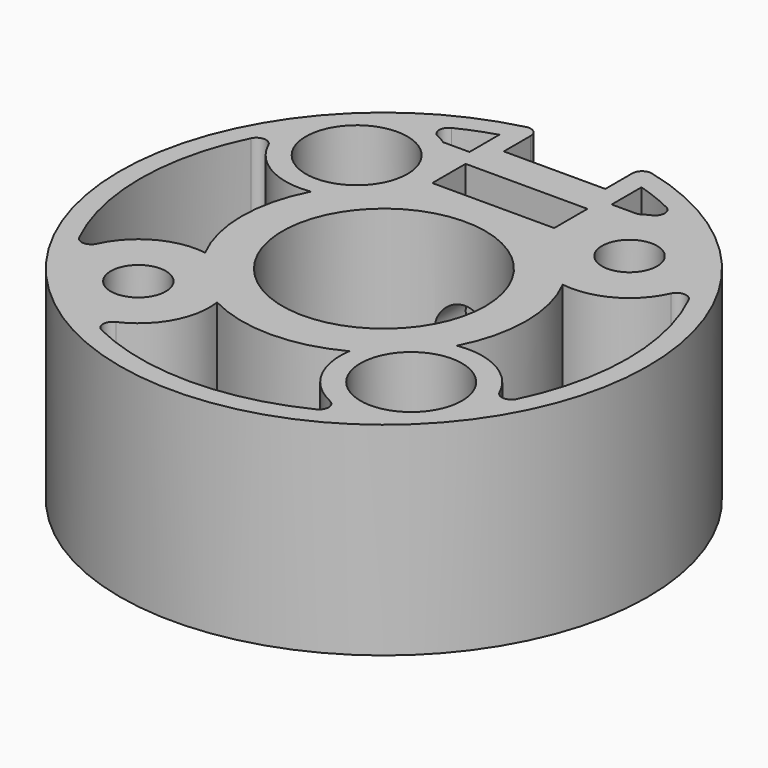
from build123d import *

# Parameters (mm, degrees)
F0_R             = 2.15265
F0_R_2           = 7.9375
F1_DEPTH         = 15.875
F2_R             = 2.15265
F3_REACH         = 43.3958636501
F6_R             = 3.96875
F7_DEPTH         = 12.7
F8_R             = 3.96875
F9_DEPTH         = 12.7
F11_DEPTH        = 15.875
F11_COPIES_COUNT = 3
F11_COPIES_ANGLE = 180
F12_R            = 2.15265
F13_REACH        = 43.3958636501
F15_DEPTH        = 15.875
F16_R            = 0.762


# Not quite as in the source:
# - a pattern or mirror of a feature is missing from the dataset's text; its kind, count and spacing are read off the source's solid


with BuildPart() as f1:
    # F0 (on Top) → F1 (new body)
    with BuildSketch(Plane.XY):
        with BuildLine():
            Line((3.96875, 16.66875), (0, 16.66875))
            Line((0, 16.66875), (-3.96875, 16.66875))
            Line((-3.96875, 16.66875), (-3.96875, 20.2522944302))
            ThreePointArc((-3.96875, 20.2522944302), (0, -20.6375), (3.96875, 20.2522944302))
            Line((3.96875, 20.2522944302), (3.96875, 16.66875))
        make_face()
        with Locations((-10.6640541438, -10.6640541438)):
            Circle(F0_R, mode=Mode.SUBTRACT)
        with Locations((10.6640541438, -10.6640541438)):
            Circle(F0_R, mode=Mode.SUBTRACT)
        with Locations((-10.6640541438, 10.6640541438)):
            Circle(F0_R, mode=Mode.SUBTRACT)
        Circle(F0_R_2, mode=Mode.SUBTRACT)
        Polygon((-4.7625, 13.928725), (0, 13.928725), (4.7625, 13.928725), (4.7625, 10.677525), (-4.7625, 10.677525), align=None, mode=Mode.SUBTRACT)
        with Locations((10.6640541438, 10.6640541438)):
            Circle(F0_R, mode=Mode.SUBTRACT)
    extrude(amount=F1_DEPTH)

    f3_end = f1.faces().sort_by_distance((-7.9375, 0, 7.9375))[0]
    # F2 (on face) → F3 (cut, up to a face of the model that its end follows)
    with BuildSketch(Plane(origin=(0, 16.66875, 0), x_dir=(-1, 0, 0), z_dir=(0, 1, 0))):
        with Locations((0, 7.9375)):
            Circle(F2_R)
    f3_long = extrude(amount=-F3_REACH, mode=Mode.PRIVATE)
    add(split(f3_long, bisect_by=f3_end, keep=Keep.ALL, mode=Mode.PRIVATE).solids().sort_by_distance((0, 16.66875, 7.9375))[0], mode=Mode.SUBTRACT)

    # F6 (on face) → F7 (cut, through all)
    with BuildSketch(Plane.XY.offset(15.875)):
        with Locations((-10.6640541438, 10.6640541438)):
            Circle(F6_R)
        with Locations((10.6640541438, -10.6640541438)):
            Circle(F6_R)
    extrude(amount=-F7_DEPTH, mode=Mode.SUBTRACT)

    # F8 (on face) → F9 (cut, through all)
    with BuildSketch(Plane(origin=(0, 0, 0), x_dir=(1, 0, 0), z_dir=(0, 0, -1))):
        with Locations((10.6640541438, -10.6640541438)):
            Circle(F8_R)
        with Locations((-10.6640541438, 10.6640541438)):
            Circle(F8_R)
    extrude(amount=-F9_DEPTH, mode=Mode.SUBTRACT)

    # F10 (on face) → F11 (cut, through all)
    with BuildSketch(Plane.XY.offset(15.875)):
        with BuildLine():
            ThreePointArc((-9.836738319, 5.1697423044), (-14.0484138573, 6.2574655095), (-16.1858200979, 10.0459806768))
            ThreePointArc((-16.1858200979, 10.0459806768), (-19.05, 0), (-16.1858200979, -10.0459806768))
            ThreePointArc((-16.1858200979, -10.0459806768), (-14.0484138573, -6.2574655095), (-9.836738319, -5.1697423044))
            ThreePointArc((-9.836738319, -5.1697423044), (-11.1125, 0), (-9.836738319, 5.1697423044))
        make_face()
    f11 = extrude(amount=-F11_DEPTH, mode=Mode.SUBTRACT)

    # F11_copies: F11 ×3 about axis
    f11_copies_axis = Axis((0, 0, 0), (0, 0, 1))
    for i in range(1, F11_COPIES_COUNT):
        add(f11.rotate(f11_copies_axis, i * F11_COPIES_ANGLE / (F11_COPIES_COUNT - 1)), mode=Mode.SUBTRACT)

    f13_end = f1.faces().sort_by_distance((-7.9375, 0, 7.9375))[0]
    # F12 (on face) → F13 (cut, up to a face of the model that its end follows)
    with BuildSketch(Plane(origin=(0, 16.66875, 0), x_dir=(-1, 0, 0), z_dir=(0, 1, 0))):
        with Locations((0, 7.9375)):
            Circle(F12_R)
    f13_long = extrude(amount=-F13_REACH, mode=Mode.PRIVATE)
    add(split(f13_long, bisect_by=f13_end, keep=Keep.TOP, mode=Mode.PRIVATE), mode=Mode.SUBTRACT)

    # F14 (on face) → F15 (cut, through all)
    with BuildSketch(Plane.XY.offset(15.875)):
        with BuildLine():
            ThreePointArc((-10.0459806768, 16.1858200979), (-8.7741608818, 15.8890151504), (-7.6067543541, 15.3035403285))
            Line((-7.6067543541, 15.3035403285), (-5.55625, 15.3035403285))
            Line((-5.55625, 15.3035403285), (-5.55625, 18.2217064497))
            ThreePointArc((-5.55625, 18.2217064497), (-7.8672491274, 17.3496078102), (-10.0459806768, 16.1858200979))
        make_face()
        with BuildLine():
            ThreePointArc((10.0459806768, 16.1858200979), (7.8672491274, 17.3496078102), (5.55625, 18.2217064497))
            Line((5.55625, 18.2217064497), (5.55625, 15.3035403285))
            Line((5.55625, 15.3035403285), (7.6067543541, 15.3035403285))
            ThreePointArc((7.6067543541, 15.3035403285), (8.7741608818, 15.8890151504), (10.0459806768, 16.1858200979))
        make_face()
    extrude(amount=-F15_DEPTH, mode=Mode.SUBTRACT)

    # F16
    f16_edges = [f1.edges().sort_by_distance(p)[0] for p in [
        (-16.18582, -10.045981, 7.9375),
        (-16.18582, 10.045981, 7.9375),
        (10.045981, 16.18582, 7.9375),
        (3.96875, 20.252294, 7.9375),
        (-3.96875, 20.252294, 7.9375),
        (-10.045981, 16.18582, 7.9375),
        (10.045981, -16.18582, 7.9375),
        (-10.045981, -16.18582, 7.9375),
        (16.18582, 10.045981, 7.9375),
        (16.18582, -10.045981, 7.9375),
    ]]
    fillet(f16_edges, radius=F16_R)


solid = f1.part
